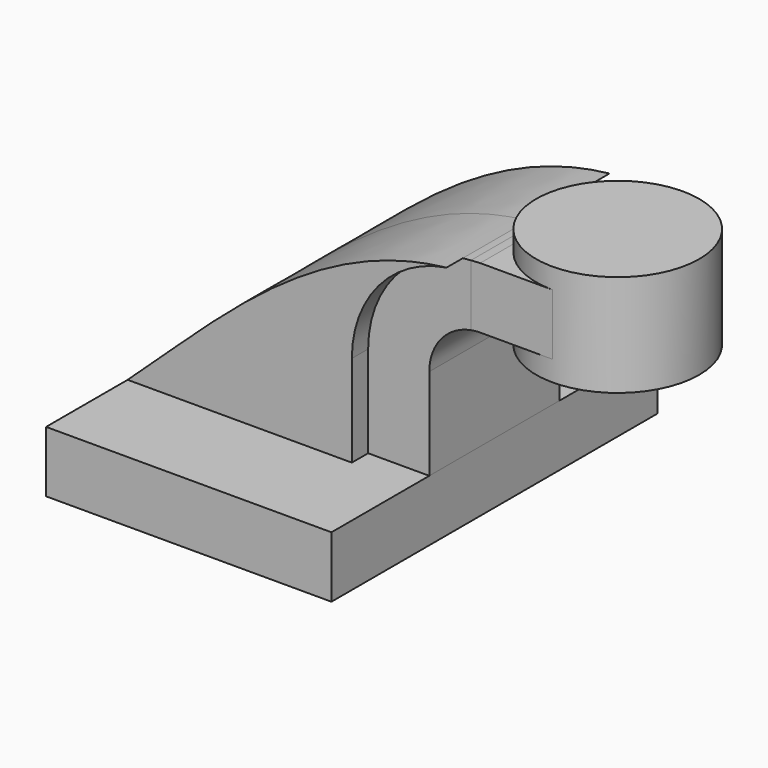
from build123d import *

# Parameters (mm, degrees)
F1_DEPTH = 63.5
F2_DEPTH = 31.75
F3_DEPTH = 25.4
F5_DEPTH = 25.4


with BuildPart() as f1:
    # F0 (on Front) → F1 (new body, symmetric)
    with BuildSketch(Plane.XZ):
        Polygon((44.45, -9.525), (44.45, 9.525), (25.4, 9.525), (-44.45, 9.525), (-44.45, -9.525), align=None)
    extrude(amount=F1_DEPTH, both=True)

    # F0 (on Front) → F2 (join, symmetric)
    with BuildSketch(Plane.XZ):
        with BuildLine():
            Line((-44.45, 9.525), (25.4, 9.525))
            Line((25.4, 9.525), (25.4, 38.1))
            ThreePointArc((25.4, 38.1), (33.7768130044, 60.7924963864), (54.8888699925, 72.5993350014))
            add(Edge.make_bspline(
                [(-44.45, 9.525), (-17.630573516, 33.748828198), (12.5933430679, 67.9708407592), (54.8888699925, 72.5993350014)],
                knots=[0, 0, 0, 0, 117.5404990535, 117.5404990535, 117.5404990535, 117.5404990535], degree=3))
        make_face()
    extrude(amount=F2_DEPTH, both=True)


with BuildPart() as f3:
    # F0 (on Front) → F3 (new body, symmetric)
    with BuildSketch(Plane.XZ):
        with BuildLine():
            Line((57.4240950841, 72.8398465542), (57.4240950841, 53.7077024468))
            ThreePointArc((57.4240950841, 53.7077024468), (58.8684031689, 53.9080343709), (60.325, 53.975))
            Line((60.325, 53.975), (82.8240950841, 53.975))
            Line((82.8240950841, 53.975), (82.8240950841, 73.025))
            Line((82.8240950841, 73.025), (60.325, 73.025))
            add(Edge.make_bspline(
                [(57.4240950841, 72.8398465542), (58.3848548691, 72.9170376368), (59.3517904465, 72.9789049543), (60.325, 73.025)],
                knots=[119.8756830341, 119.8756830341, 119.8756830341, 119.8756830341, 122.515511773, 122.515511773, 122.515511773, 122.515511773], degree=3))
        make_face()
    extrude(amount=F3_DEPTH, both=True)


with BuildPart() as f4:
    # F0 (on Front) → F4 (revolve)
    with BuildSketch(Plane.XZ):
        Polygon((82.8240950841, 53.975), (82.8240950841, 47.625), (108.2240950841, 47.625), (108.2240950841, 79.375), (82.8240950841, 79.375), (82.8240950841, 73.025), align=None)
    revolve(axis=Axis((82.8240950841, 0, 63.5), (0, 0, -1)))


with BuildPart() as f5:
    # F0 (on Front) → F5 (new body, symmetric)
    with BuildSketch(Plane.XZ):
        with BuildLine():
            Line((25.4, 9.525), (44.45, 9.525))
            Line((44.45, 9.525), (44.45, 38.1))
            ThreePointArc((44.45, 38.1), (48.1170622024, 48.2479988042), (57.4240950841, 53.7077024468))
            Line((57.4240950841, 53.7077024468), (57.4240950841, 72.8398465542))
            add(Edge.make_bspline(
                [(54.8888699925, 72.5993350014), (55.7291577038, 72.6912895677), (56.5742100798, 72.7715635718), (57.4240950841, 72.8398465542)],
                knots=[117.5404990535, 117.5404990535, 117.5404990535, 117.5404990535, 119.8756830341, 119.8756830341, 119.8756830341, 119.8756830341], degree=3))
            ThreePointArc((54.8888699925, 72.5993350014), (33.7768130044, 60.7924963864), (25.4, 38.1))
            Line((25.4, 38.1), (25.4, 9.525))
        make_face()
    extrude(amount=F5_DEPTH, both=True)


solid = Compound([f1.part, f3.part, f4.part, f5.part])
